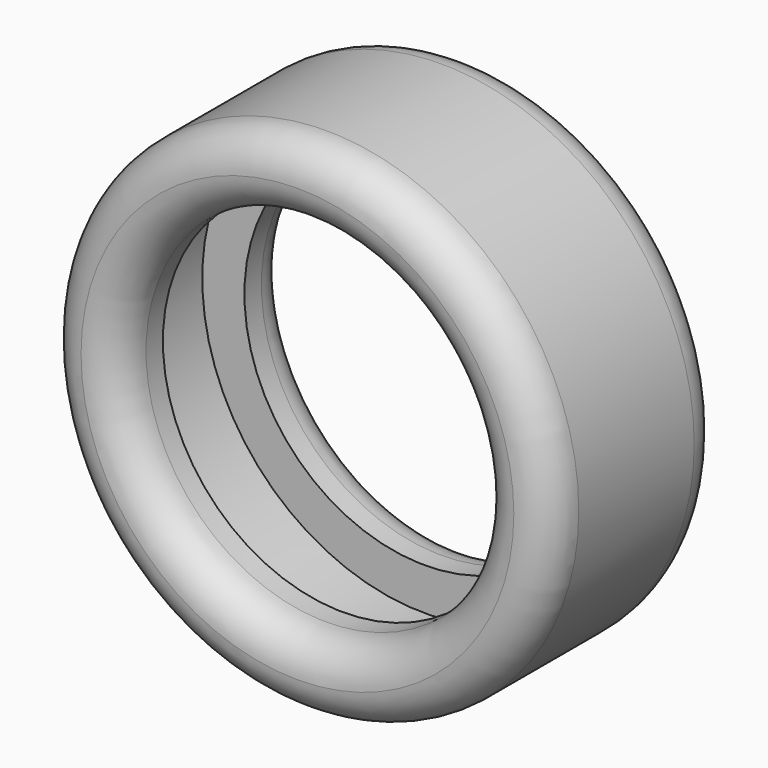
from build123d import *

# Parameters (mm, degrees)
F0_R     = 35
F0_R_2   = 25
F1_DEPTH = 15
F2_R     = 4.99999
F3_R     = 30.85
F3_R_2   = 25.79
F4_DEPTH = 7.065


# Not quite as in the source:
# - a fillet or chamfer is up to 0.001 mm smaller than in the source, because OpenCascade refuses the exact size


with BuildPart() as f1:
    # F0 (on Front) → F1 (new body, symmetric)
    with BuildSketch(Plane.XZ):
        Circle(F0_R)
        Circle(F0_R_2, mode=Mode.SUBTRACT)
    extrude(amount=F1_DEPTH, both=True)

    # F2 (radius 5 in the source; OpenCascade refuses exactly that, so slightly less here)
    f2_edges = [f1.edges().sort_by_distance(p)[0] for p in [
        (-35, -15, 0),
        (-25, -15, 0),
        (-35, 15, 0),
        (-25, 15, 0),
    ]]
    fillet(f2_edges, radius=F2_R)

    # F3 (on Front) → F4 (cut, symmetric)
    with BuildSketch(Plane.XZ):
        Circle(F3_R)
        Circle(F3_R_2, mode=Mode.SUBTRACT)
        Circle(F3_R_2)
    extrude(amount=F4_DEPTH, both=True, mode=Mode.SUBTRACT)


solid = f1.part
